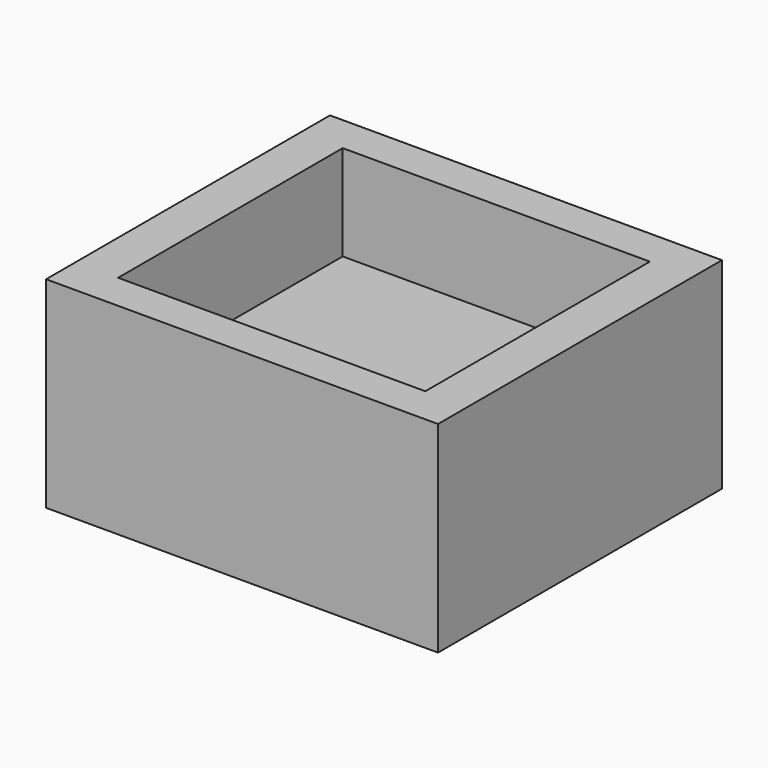
from build123d import *

# Parameters (mm, degrees)
F0_W     = 7.4
F0_H     = 6.7
F0_W_2   = 5.8
F0_H_2   = 5.3
F1_DEPTH = 1.8
F2_W     = 7.4
F2_H     = 6.7
F3_DEPTH = 2


# Not quite as in the source:
# - a feature names something its author has since deleted; it is built from what else it names


with BuildPart() as f1:
    # F0 (on Top) → F1 (new body)
    with BuildSketch(Plane.XY):
        Rectangle(F0_W, F0_H)
        Rectangle(F0_W_2, F0_H_2, mode=Mode.SUBTRACT)
    extrude(amount=F1_DEPTH)

    # F2 (on face) → F3 (join)
    with BuildSketch(Plane(origin=(0, 0, 0), x_dir=(1, 0, 0), z_dir=(0, 0, -1))):
        Rectangle(F2_W, F2_H)
    extrude(amount=F3_DEPTH)


solid = f1.part
